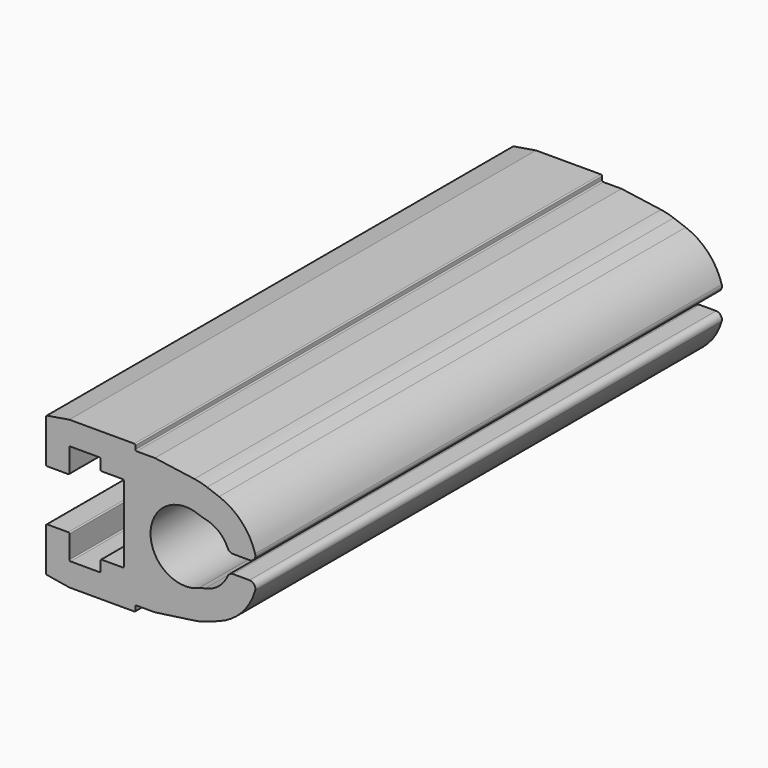
from build123d import *

# Parameters (mm, degrees)
F1_DEPTH = 150
F2_W     = 24
F2_H     = 5.125
F3_DEPTH = 0.1
F4_DEPTH = 0.1


# Not quite as in the source:
# - ends of sketch curves that miss each other by under 0.0002 mm in the source are joined


with BuildPart() as f1:
    # F0 (on Front) → F1 (new body)
    with BuildSketch(Plane.XZ):
        with BuildLine():
            Line((53.992555, -15.220268), (57.083133, -14.095389))
            ThreePointArc((57.083133, -14.095389), (62.9018568836, -10.252747544), (66.3544503107, -4.1944440905))
            ThreePointArc((66.3544503107, -4.1944440905), (66.1141142416, -2.8747683688), (64.914288, -2.275))
            Line((64.914288, -2.275), (60.670593, -2.275))
            ThreePointArc((60.670593, -2.275), (59.8472095147, -2.5211899521), (59.2941043505, -3.1789471518))
            ThreePointArc((59.2941043505, -3.1789471518), (56.9827494729, -6.2209259886), (53.52425904, -7.8441451998))
            ThreePointArc((53.52425904, -7.8441451998), (52.6431740995, -8.0626756758), (51.7855370008, -8.3602070021))
            ThreePointArc((51.7855370008, -8.3602070021), (39.452831, 0), (51.7855371982, 8.3602074972))
            ThreePointArc((51.7855371982, 8.3602074972), (52.6431743712, 8.0626765952), (53.524259133, 7.844145664))
            ThreePointArc((53.524259133, 7.844145664), (56.9827494729, 6.2209259886), (59.2941043849, 3.1789471667))
            ThreePointArc((59.2941043849, 3.1789471667), (59.8472095147, 2.5211899521), (60.670593, 2.275))
            Line((60.670593, 2.275), (64.914288, 2.275))
            ThreePointArc((64.914288, 2.275), (66.1141145297, 2.8747687527), (66.3544497778, 4.1944449353))
            ThreePointArc((66.3544497778, 4.1944449353), (62.9018565554, 10.2527478944), (57.0831331177, 14.0953893235))
            Line((57.0831331177, 14.0953893235), (53.992555, 15.220268))
            ThreePointArc((53.992555, 15.220268), (52.3736165632, 15.715360306), (50.7118440801, 16.0387645685))
            Line((50.7118440801, 16.0387645685), (40.585713, 17.465))
            Line((40.585713, 17.465), (35.885713, 17.465))
            ThreePointArc((35.885713, 17.465), (35.6735809656, 17.5528679656), (35.585713, 17.765))
            Line((35.585713, 17.765), (35.585713, 18.7))
            ThreePointArc((35.585713, 18.7), (35.4978450344, 18.9121320344), (35.285713, 19))
            Line((35.285713, 19), (18.585713, 19))
            Line((18.585713, 19), (12.836393, 18.04178))
            ThreePointArc((12.836393, 18.04178), (12.656806899, 17.9397743434), (12.585713, 17.745862))
            Line((12.585713, 17.745862), (12.585713, 6.875))
            ThreePointArc((12.585713, 6.875), (12.6735809656, 6.6628679656), (12.885713, 6.575))
            Line((12.885713, 6.575), (18.285713, 6.575))
            ThreePointArc((18.285713, 6.575), (18.4978450344, 6.6628679656), (18.585713, 6.875))
            Line((18.585713, 6.875), (18.585713, 12.7))
            ThreePointArc((18.585713, 12.7), (18.6735809656, 12.9121320344), (18.885713, 13))
            Line((18.885713, 13), (26.285713, 13))
            ThreePointArc((26.285713, 13), (26.4978450344, 12.9121320344), (26.585713, 12.7))
            Line((26.585713, 12.7), (26.585713, 10.3))
            ThreePointArc((26.585713, 10.3), (26.6735809656, 10.0878679656), (26.885713, 10))
            Line((26.885713, 10), (32.285713, 10))
            ThreePointArc((32.285713, 10), (32.4978450344, 9.9121320344), (32.585713, 9.7))
            Line((32.585713, 9.7), (32.585713, -9.7))
            ThreePointArc((32.585713, -9.7), (32.4978450344, -9.9121320344), (32.285713, -10))
            Line((32.285713, -10), (26.885713, -10))
            ThreePointArc((26.885713, -10), (26.6735809656, -10.0878679656), (26.585713, -10.3))
            Line((26.585713, -10.3), (26.585713, -12.7))
            ThreePointArc((26.585713, -12.7), (26.4978450344, -12.9121320344), (26.285713, -13))
            Line((26.285713, -13), (18.885713, -13))
            ThreePointArc((18.885713, -13), (18.6735809656, -12.9121320344), (18.585713, -12.7))
            Line((18.585713, -12.7), (18.585713, -6.875))
            ThreePointArc((18.585713, -6.875), (18.4978450344, -6.6628679656), (18.285713, -6.575))
            Line((18.285713, -6.575), (12.885713, -6.575))
            ThreePointArc((12.885713, -6.575), (12.6735809656, -6.6628679656), (12.585713, -6.875))
            Line((12.585713, -6.875), (12.585713, -17.745862))
            ThreePointArc((12.585713, -17.745862), (12.656806899, -17.9397743434), (12.8363929795, -18.0417801231))
            Line((12.8363929795, -18.0417801231), (18.585713, -19))
            Line((18.585713, -19), (35.285713, -19))
            ThreePointArc((35.285713, -19), (35.4978450344, -18.9121320344), (35.585713, -18.7))
            Line((35.585713, -18.7), (35.585713, -17.765))
            ThreePointArc((35.585713, -17.765), (35.6735809656, -17.5528679656), (35.885713, -17.465))
            Line((35.885713, -17.465), (40.585713, -17.465))
            Line((40.585713, -17.465), (50.711844, -16.038764))
            ThreePointArc((50.711844, -16.038764), (52.3736165632, -15.715360306), (53.992555, -15.220268))
        make_face()
    extrude(amount=-F1_DEPTH)

    # F2 (on face) → F3 (join)
    with BuildSketch(Plane.YZ.offset(18.585713)):
        with Locations((37.5, 9.4375)):
            Rectangle(F2_W, F2_H)
    extrude(amount=F3_DEPTH)

    # F2 (on face) → F4 (join)
    with BuildSketch(Plane.YZ.offset(18.585713)):
        with Locations((37.5, -9.4375)):
            Rectangle(F2_W, F2_H)
    extrude(amount=F4_DEPTH)


solid = f1.part
